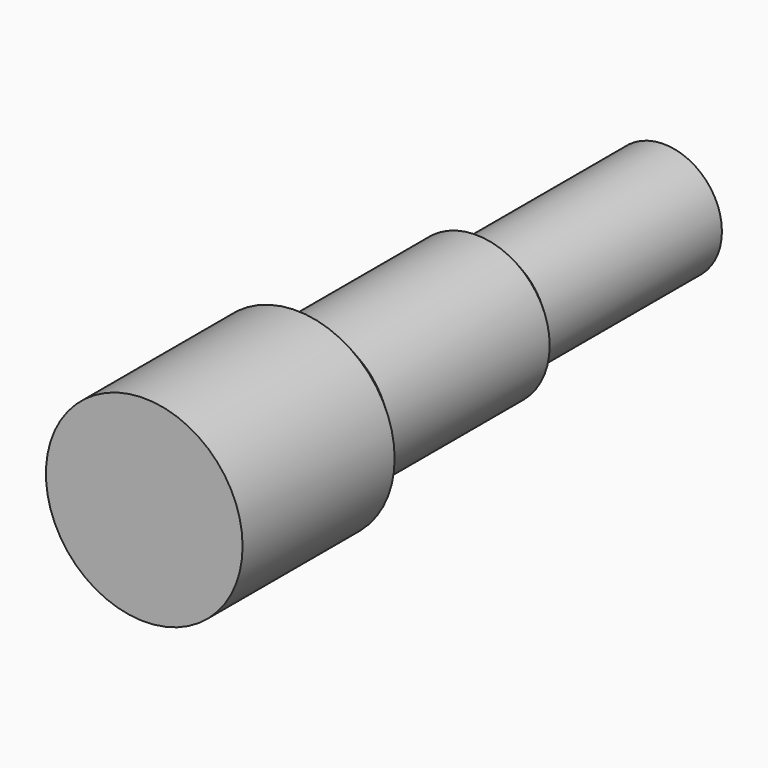
from build123d import *

# Parameters (mm, degrees)
F0_R     = 40.346618638
F1_DEPTH = 88.138
F2_SIZE  = 10.16
F3_DEPTH = 88.392
F4_SIZE  = 6.35
F5_DEPTH = 89.916


with BuildPart() as f1:
    # F0 (on Front) → F1 (new body)
    with BuildSketch(Plane.XZ):
        Circle(F0_R)
    extrude(amount=-F1_DEPTH)

    # F2
    f2_edges = [f1.edges().sort_by_distance(p)[0] for p in [
        (-40.346619, 88.138, 0),
    ]]
    chamfer(f2_edges, length=F2_SIZE)

    # F3 (add): a face of the model
    f3_faces = [f1.faces().sort_by_distance(p)[0] for p in [
        (0, 88.138, 0),
    ]]
    extrude(f3_faces, amount=F3_DEPTH)

    # F4
    f4_edges = [f1.edges().sort_by_distance(p)[0] for p in [
        (-30.186619, 176.53, 0),
    ]]
    chamfer(f4_edges, length=F4_SIZE)

    # F5 (add): a face of the model
    f5_faces = [f1.faces().sort_by_distance(p)[0] for p in [
        (0, 176.53, 0),
    ]]
    extrude(f5_faces, amount=F5_DEPTH)


solid = f1.part
